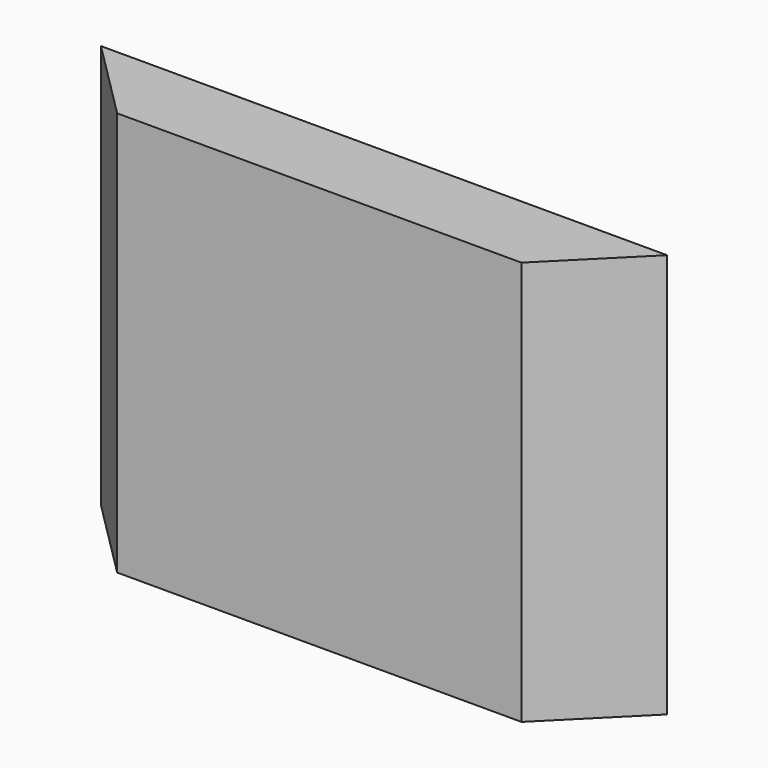
from build123d import *

# Parameters (mm, degrees)
F0_W     = 140
F0_H     = 100
F1_DEPTH = 10
F2_SIZE2 = 19.99999
F2_SIZE  = 19.99999
F3_SIZE2 = 19.99999
F3_SIZE  = 19.99999


# Not quite as in the source:
# - a fillet or chamfer is up to 0.001 mm smaller than in the source, because OpenCascade refuses the exact size


with BuildPart() as f1:
    # F0 (on Front) → F1 (new body, symmetric)
    with BuildSketch(Plane.XZ):
        with Locations((70, 50)):
            Rectangle(F0_W, F0_H)
    extrude(amount=F1_DEPTH, both=True)

    # F2 (size 20 and 20 in the source; OpenCascade refuses exactly that, so slightly less here)
    f2_edges = [f1.edges().sort_by_distance(p)[0] for p in [
        (140, -10, 50),
    ]]
    chamfer(f2_edges, length=F2_SIZE, length2=F2_SIZE2)

    # F3 (size 20 and 20 in the source; OpenCascade refuses exactly that, so slightly less here)
    f3_edges = [f1.edges().sort_by_distance(p)[0] for p in [
        (0, -10, 50),
    ]]
    chamfer(f3_edges, length=F3_SIZE, length2=F3_SIZE2)


solid = f1.part
